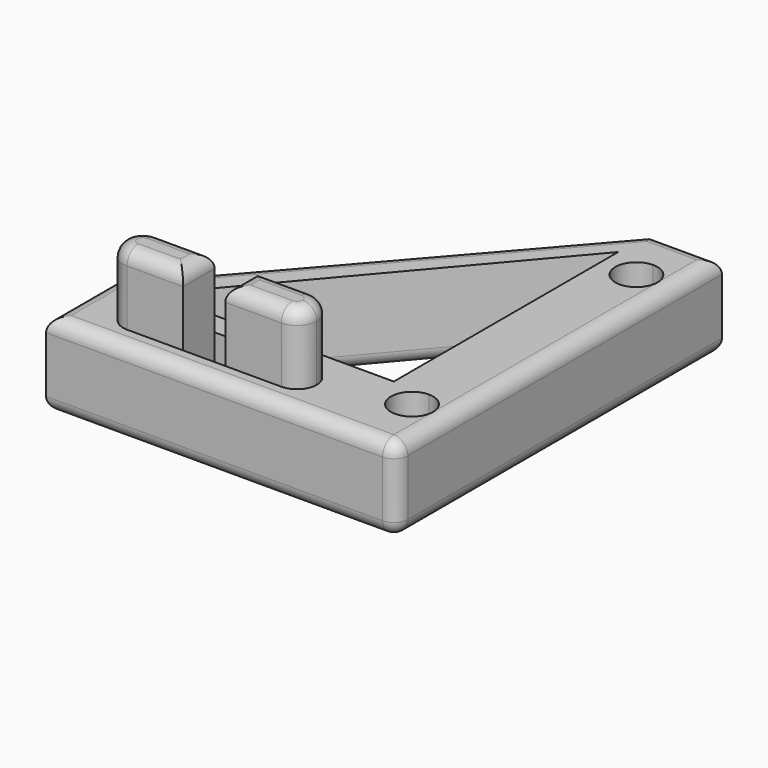
from build123d import *

# Parameters (mm, degrees)
F1_DEPTH      = 6
F2_DEPTH      = 11
F3_R          = 1
F4_T1_DEPTH   = 35.4795013083
F4_T3_DEPTH   = 11
F4_T5_DEPTH   = 26.5
F4_T7_DEPTH   = 30.5
F4_T9_DEPTH   = 10
F4_T11_DEPTH  = 3
F4_T13_DEPTH  = 2.8
F4_T15_DEPTH  = 4
F4_T17_DEPTH  = 6.5
F4_T19_DEPTH  = 7.8
F4_S23_W      = 1
F4_S23_H      = 1
F4_T24_DEPTH  = 1
F4_S29_W      = 1
F4_S29_H      = 1
F4_T30_DEPTH  = 1
F4_T36_DEPTH  = 31.2488094968
F4_T42_DEPTH  = 22.5
F4_T47_DEPTH  = 19.5
F4_T54_ANGLE  = 180
F4_T59_DEPTH  = 5.5
F4_T63_DEPTH  = 5.3
F4_T70_DEPTH  = 5.3
F4_T74_DEPTH  = 5.5
F4_T81_DEPTH  = 5.3
F4_T85_DEPTH  = 5.5
F4_T92_DEPTH  = 5.5
F4_T96_DEPTH  = 5.3
F4_T103_DEPTH = 31.2488094968
F4_T107_DEPTH = 19.5
F4_T114_DEPTH = 31.2488094968
F4_T118_DEPTH = 22.5
F4_T125_DEPTH = 25
F4_T129_DEPTH = 22


# Not quite as in the source:
# - a fillet or chamfer that OpenCascade refuses, or shapes differently, is made with other operations: its cross-section is extruded or revolved along the edge and cut away or added


with BuildPart() as f1:
    # F0 (on Top) → F1 (new body)
    with BuildSketch(Plane.XY):
        Polygon((0, 29), (-20, 6), (-17, 6), (0, 26), align=None)
        with BuildLine():
            Line((0, 3), (0, 0))
            Line((0, 0), (2.5, 0))
            Line((2.5, 0), (2.5, 3))
            ThreePointArc((2.5, 3), (1, 4.5), (2.5, 6))
            Line((2.5, 6), (2.5, 23))
            ThreePointArc((2.5, 23), (1, 24.5), (2.5, 26))
            Line((2.5, 26), (2.5, 29))
            Line((2.5, 29), (0, 29))
            Line((0, 29), (0, 26))
            Line((0, 26), (0, 6))
            Line((0, 6), (0, 3))
        make_face()
        with BuildLine():
            Line((2.5, 3), (2.5, 0))
            Line((2.5, 0), (5, 0))
            Line((5, 0), (5, 15))
            Line((5, 15), (5, 29))
            Line((5, 29), (2.5, 29))
            Line((2.5, 29), (2.5, 26))
            ThreePointArc((2.5, 26), (3.5606601718, 25.5606601718), (4, 24.5))
            ThreePointArc((4, 24.5), (3.5606601718, 23.4393398282), (2.5, 23))
            Line((2.5, 23), (2.5, 6))
            ThreePointArc((2.5, 6), (3.5606601718, 5.5606601718), (4, 4.5))
            ThreePointArc((4, 4.5), (3.5606601718, 3.4393398282), (2.5, 3))
        make_face()
        with BuildLine():
            Line((-3.1, 3), (0, 3))
            Line((0, 3), (0, 6))
            Line((0, 6), (-17, 6))
            Line((-17, 6), (-20, 6))
            Line((-20, 6), (-20, 3))
            Line((-20, 3), (-16.9, 3))
            ThreePointArc((-16.9, 3), (-16.4899494937, 3.9899494937), (-15.5, 4.4))
            Line((-15.5, 4.4), (-11.5, 4.4))
            Line((-11.5, 4.4), (-10, 4.4))
            Line((-10, 4.4), (-8.5, 4.4))
            Line((-8.5, 4.4), (-4.5, 4.4))
            ThreePointArc((-4.5, 4.4), (-3.5100505063, 3.9899494937), (-3.1, 3))
        make_face()
        with BuildLine():
            Line((-20, 0), (0, 0))
            Line((0, 0), (0, 3))
            Line((0, 3), (-3.1, 3))
            ThreePointArc((-3.1, 3), (-3.5100505063, 2.0100505063), (-4.5, 1.6))
            Line((-4.5, 1.6), (-8.5, 1.6))
            Line((-8.5, 1.6), (-10, 1.6))
            Line((-10, 1.6), (-11.5, 1.6))
            Line((-11.5, 1.6), (-15.5, 1.6))
            ThreePointArc((-15.5, 1.6), (-16.4899494937, 2.0100505063), (-16.9, 3))
            Line((-16.9, 3), (-20, 3))
            Line((-20, 3), (-20, 0))
        make_face()
    extrude(amount=F1_DEPTH)

    # F0 (on Top) → F2 (join)
    with BuildSketch(Plane.XY):
        with BuildLine():
            Line((-14.1, 3), (-16.9, 3))
            ThreePointArc((-16.9, 3), (-16.4899494937, 2.0100505063), (-15.5, 1.6))
            ThreePointArc((-15.5, 1.6), (-14.5100505063, 2.0100505063), (-14.1, 3))
        make_face()
        with BuildLine():
            ThreePointArc((-4.5, 1.6), (-5.4899494937, 2.0100505063), (-5.9, 3))
            Line((-5.9, 3), (-8.5, 3))
            Line((-8.5, 3), (-8.5, 1.6))
            Line((-8.5, 1.6), (-4.5, 1.6))
        make_face()
        with BuildLine():
            Line((-11.5, 3), (-14.1, 3))
            ThreePointArc((-14.1, 3), (-14.5100505063, 2.0100505063), (-15.5, 1.6))
            Line((-15.5, 1.6), (-11.5, 1.6))
            Line((-11.5, 1.6), (-11.5, 3))
        make_face()
        with BuildLine():
            ThreePointArc((-15.5, 4.4), (-14.5100505063, 3.9899494937), (-14.1, 3))
            Line((-14.1, 3), (-11.5, 3))
            Line((-11.5, 3), (-11.5, 4.4))
            Line((-11.5, 4.4), (-15.5, 4.4))
        make_face()
        with BuildLine():
            Line((-8.5, 3), (-5.9, 3))
            ThreePointArc((-5.9, 3), (-5.4899494937, 3.9899494937), (-4.5, 4.4))
            Line((-4.5, 4.4), (-8.5, 4.4))
            Line((-8.5, 4.4), (-8.5, 3))
        make_face()
        with BuildLine():
            Line((-5.9, 3), (-3.1, 3))
            ThreePointArc((-3.1, 3), (-3.5100505063, 3.9899494937), (-4.5, 4.4))
            ThreePointArc((-4.5, 4.4), (-5.4899494937, 3.9899494937), (-5.9, 3))
        make_face()
        with BuildLine():
            ThreePointArc((-4.5, 1.6), (-3.5100505063, 2.0100505063), (-3.1, 3))
            Line((-3.1, 3), (-5.9, 3))
            ThreePointArc((-5.9, 3), (-5.4899494937, 2.0100505063), (-4.5, 1.6))
        make_face()
        with BuildLine():
            ThreePointArc((-15.5, 4.4), (-16.4899494937, 3.9899494937), (-16.9, 3))
            Line((-16.9, 3), (-14.1, 3))
            ThreePointArc((-14.1, 3), (-14.5100505063, 3.9899494937), (-15.5, 4.4))
        make_face()
    extrude(amount=F2_DEPTH)

    # F3
    f3_edges = [f1.edges().sort_by_distance(p)[0] for p in [
        (-6.5, 4.4, 11),
        (-8.5, 3, 11),
        (-6.5, 1.6, 11),
        (-3.1, 3, 11),
    ]]
    fillet(f3_edges, radius=F3_R)

    # F4: fillet of radius 1 on 24 edges, made by hand

    # F4_s2 → F4_t1 (cut)
    with BuildSketch(Plane(origin=(15.9999731598, 18.3999691337, 0), x_dir=(0, 0, 1), z_dir=(-0.6561787149, -0.7546055222, 0))):
        with BuildLine():
            ThreePointArc((0, 18.0291827328), (0.2928932188, 18.736289514), (1, 19.0291827328))
            Line((1, 19.0291827328), (0, 19.0291827328))
            Line((0, 19.0291827328), (0, 18.0291827328))
        make_face()
        with BuildLine():
            ThreePointArc((6, 18.0291827328), (5.7071067812, 18.736289514), (5, 19.0291827328))
            Line((5, 19.0291827328), (6, 19.0291827328))
            Line((6, 19.0291827328), (6, 18.0291827328))
        make_face()
    extrude(amount=F4_T1_DEPTH, mode=Mode.SUBTRACT)

    # F4_s4 → F4_t3 (cut)
    with BuildSketch(Plane.XZ.offset(-8.5)):
        with BuildLine():
            ThreePointArc((-19, 0), (-19.7071067812, 0.2928932188), (-20, 1))
            Line((-20, 1), (-20, 0))
            Line((-20, 0), (-19, 0))
        make_face()
        with BuildLine():
            ThreePointArc((-19, 6), (-19.7071067812, 5.7071067812), (-20, 5))
            Line((-20, 5), (-20, 6))
            Line((-20, 6), (-19, 6))
        make_face()
    extrude(amount=F4_T3_DEPTH, mode=Mode.SUBTRACT)

    # F4_s6 → F4_t5 (cut)
    with BuildSketch(Plane.YZ.offset(-22.5)):
        with BuildLine():
            ThreePointArc((1, 0), (0.2928932188, 0.2928932188), (0, 1))
            Line((0, 1), (0, 0))
            Line((0, 0), (1, 0))
        make_face()
        with BuildLine():
            ThreePointArc((1, 6), (0.2928932188, 5.7071067812), (0, 5))
            Line((0, 5), (0, 6))
            Line((0, 6), (1, 6))
        make_face()
    extrude(amount=F4_T5_DEPTH, mode=Mode.SUBTRACT)

    # F4_s8 → F4_t7 (cut)
    with BuildSketch(Plane.XZ.offset(-31.5)):
        with BuildLine():
            ThreePointArc((4, 0), (4.7071067812, 0.2928932188), (5, 1))
            Line((5, 1), (5, 0))
            Line((5, 0), (4, 0))
        make_face()
        with BuildLine():
            ThreePointArc((4, 6), (4.7071067812, 5.7071067812), (5, 5))
            Line((5, 5), (5, 6))
            Line((5, 6), (4, 6))
        make_face()
    extrude(amount=F4_T7_DEPTH, mode=Mode.SUBTRACT)

    # F4_s10 → F4_t9 (cut)
    with BuildSketch(Plane.YZ.offset(-2.5)):
        with BuildLine():
            ThreePointArc((28, 0), (28.7071067812, 0.2928932188), (29, 1))
            Line((29, 1), (29, 0))
            Line((29, 0), (28, 0))
        make_face()
        with BuildLine():
            ThreePointArc((28, 6), (28.7071067812, 5.7071067812), (29, 5))
            Line((29, 5), (29, 6))
            Line((29, 6), (28, 6))
        make_face()
    extrude(amount=F4_T9_DEPTH, mode=Mode.SUBTRACT)

    # F4_s12 → F4_t11 (cut)
    with BuildSketch(Plane.YZ.offset(-11.5)):
        with BuildLine():
            ThreePointArc((4.4, 1), (4.6928932188, 0.2928932188), (5.4, 0))
            Line((5.4, 0), (4.4, 0))
            Line((4.4, 0), (4.4, 1))
        make_face()
        with BuildLine():
            ThreePointArc((0.6, 0), (1.3071067812, 0.2928932188), (1.6, 1))
            Line((1.6, 1), (1.6, 0))
            Line((1.6, 0), (0.6, 0))
        make_face()
    extrude(amount=F4_T11_DEPTH, mode=Mode.SUBTRACT)

    # F4_s14 → F4_t13 (cut)
    with BuildSketch(Plane.XZ.offset(-4.4)):
        with BuildLine():
            ThreePointArc((-8.5, 1), (-8.2071067812, 0.2928932188), (-7.5, 0))
            Line((-7.5, 0), (-8.5, 0))
            Line((-8.5, 0), (-8.5, 1))
        make_face()
        with BuildLine():
            ThreePointArc((-12.5, 0), (-11.7928932188, 0.2928932188), (-11.5, 1))
            Line((-11.5, 1), (-11.5, 0))
            Line((-11.5, 0), (-12.5, 0))
        make_face()
    extrude(amount=F4_T13_DEPTH, mode=Mode.SUBTRACT)

    # F4_s16 → F4_t15 (cut)
    with BuildSketch(Plane.XY.offset(1)):
        with BuildLine():
            ThreePointArc((4, 0), (4.7071067812, 0.2928932188), (5, 1))
            Line((5, 1), (5, 0))
            Line((5, 0), (4, 0))
        make_face()
    extrude(amount=F4_T15_DEPTH, mode=Mode.SUBTRACT)

    # F4_s18 → F4_t17 (cut)
    with BuildSketch(Plane.YZ.offset(-15.5)):
        with BuildLine():
            ThreePointArc((4.4, 10), (4.1071067812, 10.7071067812), (3.4, 11))
            Line((3.4, 11), (4.4, 11))
            Line((4.4, 11), (4.4, 10))
        make_face()
        with BuildLine():
            ThreePointArc((1.6, 10), (1.8928932188, 10.7071067812), (2.6, 11))
            Line((2.6, 11), (1.6, 11))
            Line((1.6, 11), (1.6, 10))
        make_face()
    extrude(amount=F4_T17_DEPTH, mode=Mode.SUBTRACT)

    # F4_s20 → F4_t19 (cut)
    with BuildSketch(Plane.XZ.offset(-6.9)):
        with BuildLine():
            ThreePointArc((-11.5, 10), (-11.7928932188, 10.7071067812), (-12.5, 11))
            Line((-12.5, 11), (-11.5, 11))
            Line((-11.5, 11), (-11.5, 10))
        make_face()
    extrude(amount=F4_T19_DEPTH, mode=Mode.SUBTRACT)


with BuildPart() as f4_tool22:
    # F4_s23 → F4_t24 (new body)
    with BuildSketch(Plane.XY.offset(1)):
        with Locations((4.5, 0.5)):
            Rectangle(F4_S23_W, F4_S23_H)
    extrude(amount=-F4_T24_DEPTH)

    # F4_s25 → F4_t26 (revolve, cut)
    with BuildSketch(Plane(origin=(4, 1, 1), x_dir=(-0.7071067812, 0.7071067812, 0), z_dir=(-0.7071067812, -0.7071067812, 0))):
        with BuildLine():
            ThreePointArc((0, -1), (1, 0), (0, 1))
            Line((0, 1), (0, -1))
        make_face()
    revolve(axis=Axis((4, 1, 1), (0, 0, -1)), mode=Mode.SUBTRACT)


with BuildPart() as f1_1:
    add(f1.part)

    # F4_t21: cut F4_tool22
    add(f4_tool22.part, mode=Mode.SUBTRACT)


with BuildPart() as f4_tool28:
    # F4_s29 → F4_t30 (new body)
    with BuildSketch(Plane.XY.offset(5)):
        with Locations((4.5, 0.5)):
            Rectangle(F4_S29_W, F4_S29_H)
    extrude(amount=F4_T30_DEPTH)

    # F4_s31 → F4_t32 (revolve, cut)
    with BuildSketch(Plane(origin=(4, 1, 5), x_dir=(-0.7071067812, 0.7071067812, 0), z_dir=(0.7071067812, 0.7071067812, 0))):
        with BuildLine():
            ThreePointArc((0, -1), (1, 0), (0, 1))
            Line((0, 1), (0, -1))
        make_face()
    revolve(axis=Axis((4, 1, 5), (0, 0, 1)), mode=Mode.SUBTRACT)


with BuildPart() as f1_2:
    add(f1_1.part)

    # F4_t27: cut F4_tool28
    add(f4_tool28.part, mode=Mode.SUBTRACT)


with BuildPart() as f4_tool34:
    # F4_s35 → F4_t36 (new body)
    with BuildSketch(Plane(origin=(-5.788932371, -6.8105086718, 0), x_dir=(0, 0, 1), z_dir=(0.6476484201, 0.7619393178, 0))):
        with BuildLine():
            ThreePointArc((0, -17.8388589225), (0.2928932188, -17.1317521413), (1, -16.8388589225))
            Line((1, -16.8388589225), (0, -16.8388589225))
            Line((0, -16.8388589225), (0, -17.8388589225))
        make_face()
    extrude(amount=F4_T36_DEPTH)

    split(bisect_by=Plane.XZ.offset(-6), keep=Keep.BOTTOM)

    split(bisect_by=Plane.YZ, keep=Keep.BOTTOM)


with BuildPart() as f1_3:
    add(f1_2.part)

    # F4_t33: cut F4_tool34
    add(f4_tool34.part, mode=Mode.SUBTRACT)


with BuildPart() as f4_tool40:
    # F4_s41 → F4_t42 (new body)
    with BuildSketch(Plane.XZ.offset(-28.5)):
        with BuildLine():
            ThreePointArc((1, 0), (0.2928932188, 0.2928932188), (0, 1))
            Line((0, 1), (0, 0))
            Line((0, 0), (1, 0))
        make_face()
    extrude(amount=F4_T42_DEPTH)

    split(bisect_by=Plane(origin=(-12.8301886792, 10.9056603774, 0), x_dir=(0, 0, 1), z_dir=(0.7619393178, -0.6476484201, 0)), keep=Keep.TOP)


with BuildPart() as f1_4:
    add(f1_3.part)

    # F4_t39: cut F4_tool40
    add(f4_tool40.part, mode=Mode.SUBTRACT)


with BuildPart() as f4_tool45:
    # F4_s46 → F4_t47 (new body)
    with BuildSketch(Plane.YZ):
        with BuildLine():
            ThreePointArc((5, 0), (5.7071067812, 0.2928932188), (6, 1))
            Line((6, 1), (6, 0))
            Line((6, 0), (5, 0))
        make_face()
    extrude(amount=-F4_T47_DEPTH)

    split(bisect_by=Plane(origin=(-12.8301886792, 10.9056603774, 0), x_dir=(0, 0, 1), z_dir=(0.7619393178, -0.6476484201, 0)), keep=Keep.TOP)


with BuildPart() as f1_5:
    add(f1_4.part)

    # F4_t44: cut F4_tool45
    add(f4_tool45.part, mode=Mode.SUBTRACT)

    # F4_s49 → F4_t50 (revolve, cut)
    with BuildSketch(Plane.YZ.offset(2.5)):
        with BuildLine():
            ThreePointArc((7, 0), (6.2928932188, 0.2928932188), (6, 1))
            Line((6, 1), (6, 0))
            Line((6, 0), (7, 0))
        make_face()
    revolve(axis=Axis((2.5, 4.5, 0), (0, 0, -1)), mode=Mode.SUBTRACT)

    # F4_s51 → F4_t52 (revolve, cut)
    with BuildSketch(Plane.YZ.offset(2.5)):
        with BuildLine():
            ThreePointArc((27, 0), (26.2928932188, 0.2928932188), (26, 1))
            Line((26, 1), (26, 0))
            Line((26, 0), (27, 0))
        make_face()
    revolve(axis=Axis((2.5, 24.5, 0), (0, 0, -1)), mode=Mode.SUBTRACT)

    # F4_s53 → F4_t54 (revolve, cut)
    with BuildSketch(Plane.YZ.offset(-15.5)):
        with BuildLine():
            ThreePointArc((4.4, 10), (4.1071067812, 10.7071067812), (3.4, 11))
            Line((3.4, 11), (4.4, 11))
            Line((4.4, 11), (4.4, 10))
        make_face()
    revolve(axis=Axis((-15.5, 3, 11), (0, 0, 1)), revolution_arc=F4_T54_ANGLE, mode=Mode.SUBTRACT)


with BuildPart() as f4_tool57:
    # F4_s58 → F4_t59 (new body)
    with BuildSketch(Plane.YZ.offset(-14)):
        with BuildLine():
            ThreePointArc((4.4, 1), (4.6928932188, 0.2928932188), (5.4, 0))
            Line((5.4, 0), (4.4, 0))
            Line((4.4, 0), (4.4, 1))
        make_face()
    extrude(amount=F4_T59_DEPTH)

    split(bisect_by=Plane.YZ.offset(-11.5), keep=Keep.BOTTOM)


with BuildPart() as f4_tool61:
    # F4_s62 → F4_t63 (new body)
    with BuildSketch(Plane.XZ.offset(-1.6)):
        with BuildLine():
            ThreePointArc((-12.5, 0), (-11.7928932188, 0.2928932188), (-11.5, 1))
            Line((-11.5, 1), (-11.5, 0))
            Line((-11.5, 0), (-12.5, 0))
        make_face()
    extrude(amount=-F4_T63_DEPTH)

    split(bisect_by=Plane.XZ.offset(-4.4), keep=Keep.BOTTOM)


with BuildPart() as f4_tool57_1:
    add(f4_tool57.part)

    # F4_t65: intersect F4_tool61
    add(f4_tool61.part, mode=Mode.INTERSECT)


with BuildPart() as f1_6:
    add(f1_5.part)

    # F4_t55: cut F4_tool57
    add(f4_tool57_1.part, mode=Mode.SUBTRACT)


with BuildPart() as f4_tool68:
    # F4_s69 → F4_t70 (new body)
    with BuildSketch(Plane.XZ.offset(-6.9)):
        with BuildLine():
            ThreePointArc((-8.5, 1), (-8.2071067812, 0.2928932188), (-7.5, 0))
            Line((-7.5, 0), (-8.5, 0))
            Line((-8.5, 0), (-8.5, 1))
        make_face()
    extrude(amount=F4_T70_DEPTH)

    split(bisect_by=Plane.XZ.offset(-4.4), keep=Keep.BOTTOM)


with BuildPart() as f4_tool72:
    # F4_s73 → F4_t74 (new body)
    with BuildSketch(Plane.YZ.offset(-11.5)):
        with BuildLine():
            ThreePointArc((4.4, 1), (4.6928932188, 0.2928932188), (5.4, 0))
            Line((5.4, 0), (4.4, 0))
            Line((4.4, 0), (4.4, 1))
        make_face()
    extrude(amount=F4_T74_DEPTH)

    split(bisect_by=Plane.YZ.offset(-8.5), keep=Keep.TOP)


with BuildPart() as f4_tool68_1:
    add(f4_tool68.part)

    # F4_t76: intersect F4_tool72
    add(f4_tool72.part, mode=Mode.INTERSECT)


with BuildPart() as f1_7:
    add(f1_6.part)

    # F4_t66: cut F4_tool68
    add(f4_tool68_1.part, mode=Mode.SUBTRACT)


with BuildPart() as f4_tool79:
    # F4_s80 → F4_t81 (new body)
    with BuildSketch(Plane.XZ.offset(-4.4)):
        with BuildLine():
            ThreePointArc((-8.5, 1), (-8.2071067812, 0.2928932188), (-7.5, 0))
            Line((-7.5, 0), (-8.5, 0))
            Line((-8.5, 0), (-8.5, 1))
        make_face()
    extrude(amount=F4_T81_DEPTH)

    split(bisect_by=Plane.XZ.offset(-1.6), keep=Keep.TOP)


with BuildPart() as f4_tool83:
    # F4_s84 → F4_t85 (new body)
    with BuildSketch(Plane.YZ.offset(-6)):
        with BuildLine():
            ThreePointArc((0.6, 0), (1.3071067812, 0.2928932188), (1.6, 1))
            Line((1.6, 1), (1.6, 0))
            Line((1.6, 0), (0.6, 0))
        make_face()
    extrude(amount=-F4_T85_DEPTH)

    split(bisect_by=Plane.YZ.offset(-8.5), keep=Keep.TOP)


with BuildPart() as f4_tool79_1:
    add(f4_tool79.part)

    # F4_t87: intersect F4_tool83
    add(f4_tool83.part, mode=Mode.INTERSECT)


with BuildPart() as f1_8:
    add(f1_7.part)

    # F4_t77: cut F4_tool79
    add(f4_tool79_1.part, mode=Mode.SUBTRACT)


with BuildPart() as f4_tool90:
    # F4_s91 → F4_t92 (new body)
    with BuildSketch(Plane.YZ.offset(-8.5)):
        with BuildLine():
            ThreePointArc((0.6, 0), (1.3071067812, 0.2928932188), (1.6, 1))
            Line((1.6, 1), (1.6, 0))
            Line((1.6, 0), (0.6, 0))
        make_face()
    extrude(amount=-F4_T92_DEPTH)

    split(bisect_by=Plane.YZ.offset(-11.5), keep=Keep.BOTTOM)


with BuildPart() as f4_tool94:
    # F4_s95 → F4_t96 (new body)
    with BuildSketch(Plane.XZ.offset(0.9)):
        with BuildLine():
            ThreePointArc((-12.5, 0), (-11.7928932188, 0.2928932188), (-11.5, 1))
            Line((-11.5, 1), (-11.5, 0))
            Line((-11.5, 0), (-12.5, 0))
        make_face()
    extrude(amount=-F4_T96_DEPTH)

    split(bisect_by=Plane.XZ.offset(-1.6), keep=Keep.TOP)


with BuildPart() as f4_tool90_1:
    add(f4_tool90.part)

    # F4_t98: intersect F4_tool94
    add(f4_tool94.part, mode=Mode.INTERSECT)


with BuildPart() as f1_9:
    add(f1_8.part)

    # F4_t88: cut F4_tool90
    add(f4_tool90_1.part, mode=Mode.SUBTRACT)


with BuildPart() as f4_tool101:
    # F4_s102 → F4_t103 (new body)
    with BuildSketch(Plane(origin=(-5.788932371, -6.8105086718, 0), x_dir=(0, 0, 1), z_dir=(0.6476484201, 0.7619393178, 0))):
        with BuildLine():
            ThreePointArc((0, -17.8388589225), (0.2928932188, -17.1317521413), (1, -16.8388589225))
            Line((1, -16.8388589225), (0, -16.8388589225))
            Line((0, -16.8388589225), (0, -17.8388589225))
        make_face()
    extrude(amount=F4_T103_DEPTH)

    split(bisect_by=Plane.XZ.offset(-6), keep=Keep.TOP)


with BuildPart() as f4_tool105:
    # F4_s106 → F4_t107 (new body)
    with BuildSketch(Plane.YZ):
        with BuildLine():
            ThreePointArc((5, 0), (5.7071067812, 0.2928932188), (6, 1))
            Line((6, 1), (6, 0))
            Line((6, 0), (5, 0))
        make_face()
    extrude(amount=-F4_T107_DEPTH)

    split(bisect_by=Plane(origin=(-12.8301886792, 10.9056603774, 0), x_dir=(0, 0, 1), z_dir=(-0.7619393178, 0.6476484201, 0)), keep=Keep.TOP)


with BuildPart() as f4_tool101_1:
    add(f4_tool101.part)

    # F4_t109: intersect F4_tool105
    add(f4_tool105.part, mode=Mode.INTERSECT)


with BuildPart() as f1_10:
    add(f1_9.part)

    # F4_t99: cut F4_tool101
    add(f4_tool101_1.part, mode=Mode.SUBTRACT)


with BuildPart() as f4_tool112:
    # F4_s113 → F4_t114 (new body)
    with BuildSketch(Plane(origin=(-5.788932371, -6.8105086718, 0), x_dir=(0, 0, 1), z_dir=(0.6476484201, 0.7619393178, 0))):
        with BuildLine():
            ThreePointArc((0, -17.8388589225), (0.2928932188, -17.1317521413), (1, -16.8388589225))
            Line((1, -16.8388589225), (0, -16.8388589225))
            Line((0, -16.8388589225), (0, -17.8388589225))
        make_face()
    extrude(amount=F4_T114_DEPTH)

    split(bisect_by=Plane.YZ, keep=Keep.TOP)


with BuildPart() as f4_tool116:
    # F4_s117 → F4_t118 (new body)
    with BuildSketch(Plane.XZ.offset(-28.5)):
        with BuildLine():
            ThreePointArc((1, 0), (0.2928932188, 0.2928932188), (0, 1))
            Line((0, 1), (0, 0))
            Line((0, 0), (1, 0))
        make_face()
    extrude(amount=F4_T118_DEPTH)

    split(bisect_by=Plane(origin=(-12.8301886792, 10.9056603774, 0), x_dir=(0, 0, 1), z_dir=(-0.7619393178, 0.6476484201, 0)), keep=Keep.TOP)


with BuildPart() as f4_tool112_1:
    add(f4_tool112.part)

    # F4_t120: intersect F4_tool116
    add(f4_tool116.part, mode=Mode.INTERSECT)


with BuildPart() as f1_11:
    add(f1_10.part)

    # F4_t110: cut F4_tool112
    add(f4_tool112_1.part, mode=Mode.SUBTRACT)


with BuildPart() as f4_tool123:
    # F4_s124 → F4_t125 (new body)
    with BuildSketch(Plane.XZ.offset(-28.5)):
        with BuildLine():
            ThreePointArc((1, 0), (0.2928932188, 0.2928932188), (0, 1))
            Line((0, 1), (0, 0))
            Line((0, 0), (1, 0))
        make_face()
    extrude(amount=F4_T125_DEPTH)

    split(bisect_by=Plane.XZ.offset(-6), keep=Keep.TOP)


with BuildPart() as f4_tool127:
    # F4_s128 → F4_t129 (new body)
    with BuildSketch(Plane.YZ.offset(2.5)):
        with BuildLine():
            ThreePointArc((5, 0), (5.7071067812, 0.2928932188), (6, 1))
            Line((6, 1), (6, 0))
            Line((6, 0), (5, 0))
        make_face()
    extrude(amount=-F4_T129_DEPTH)

    split(bisect_by=Plane.YZ, keep=Keep.TOP)


with BuildPart() as f4_tool123_1:
    add(f4_tool123.part)

    # F4_t131: intersect F4_tool127
    add(f4_tool127.part, mode=Mode.INTERSECT)


with BuildPart() as f1_12:
    add(f1_11.part)

    # F4_t121: cut F4_tool123
    add(f4_tool123_1.part, mode=Mode.SUBTRACT)


solid = f1_12.part
